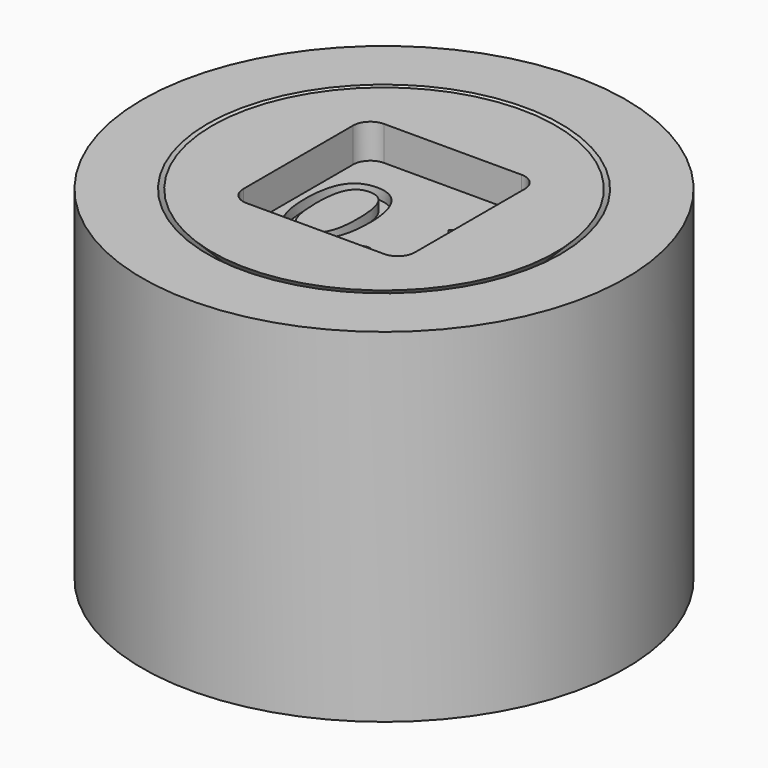
from build123d import *

# Parameters (mm, degrees)
F4_DEPTH     = 1
F5_TEXT_SIZE = 3.9945075521
F6_DEPTH     = 1.3


# Not quite as in the source:
# - Text() gives the source's letters only with a copy of the font that has no kerning and outlines rounded to 1/6400 em; it was checked with that copy


with BuildPart() as f1:
    # F0 (on Front) → F1 (revolve)
    with BuildSketch(Plane.XZ):
        with BuildLine():
            Line((-5, 0), (0, 0))
            Line((0, 0), (0, 10))
            Line((0, 10), (-5, 10))
            Line((-5, 10), (-2.7928932188, 7.7928932188))
            ThreePointArc((-2.7928932188, 7.7928932188), (-2.5761204675, 7.46846987), (-2.5, 7.0857864376))
            Line((-2.5, 7.0857864376), (-2.5, 2.9142135624))
            ThreePointArc((-2.5, 2.9142135624), (-2.5761204675, 2.53153013), (-2.7928932188, 2.2071067812))
            Line((-2.7928932188, 2.2071067812), (-5, 0))
        make_face()
    revolve(axis=Axis((0, 0, 5), (0, 0, 1)))

    # F3 (on face) → F4 (cut)
    with BuildSketch(Plane.XY.offset(10)):
        with BuildLine():
            Line((2, 2.5), (-2, 2.5))
            ThreePointArc((-2, 2.5), (-2.3535533906, 2.3535533906), (-2.5, 2))
            Line((-2.5, 2), (-2.5, -2))
            ThreePointArc((-2.5, -2), (-2.3535533906, -2.3535533906), (-2, -2.5))
            Line((-2, -2.5), (2, -2.5))
            ThreePointArc((2, -2.5), (2.3535533906, -2.3535533906), (2.5, -2))
            Line((2.5, -2), (2.5, 2))
            ThreePointArc((2.5, 2), (2.3535533906, 2.3535533906), (2, 2.5))
        make_face()
    extrude(amount=-F4_DEPTH, mode=Mode.SUBTRACT)

    # F5 (on offset) → F6 (cut)
    with BuildSketch(Plane.XY.offset(10)):
        with Locations((-2.5, -1.4380227188)):
            Text('0.1', F5_TEXT_SIZE, font='Open Sans', text_align=(TextAlign.LEFT, TextAlign.BOTTOM))
    extrude(amount=-F6_DEPTH, mode=Mode.SUBTRACT)


with BuildPart() as f1b:
    # F0 (on Front) → F1, piece 2 (revolve)
    with BuildSketch(Plane.XZ):
        with BuildLine():
            Line((-7.0414213562, 10), (-7.0414213562, 0))
            Line((-7.0414213562, 0), (-5.1414213562, 0))
            Line((-5.1414213562, 0), (-2.8928932188, 2.2485281374))
            ThreePointArc((-2.8928932188, 2.2485281374), (-2.6761204675, 2.5729514862), (-2.6, 2.9556349186))
            Line((-2.6, 2.9556349186), (-2.6, 7.0443650814))
            ThreePointArc((-2.6, 7.0443650814), (-2.6761204675, 7.4270485138), (-2.8928932188, 7.7514718626))
            Line((-2.8928932188, 7.7514718626), (-5.1414213562, 10))
            Line((-5.1414213562, 10), (-7.0414213562, 10))
        make_face()
    revolve(axis=Axis((0, 0, 5), (0, 0, 1)))


solid = Compound([f1.part, f1b.part])
